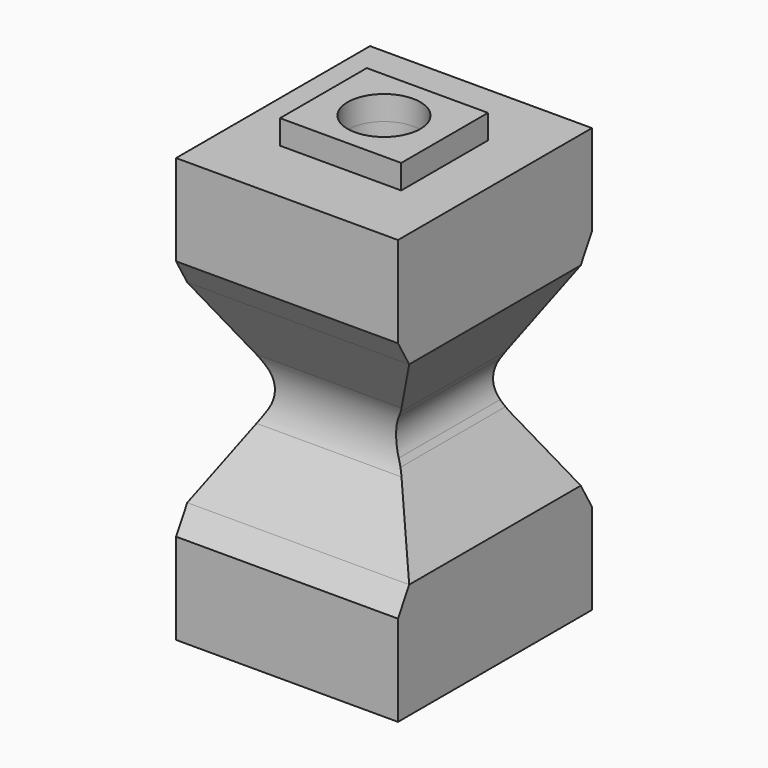
from build123d import *

# Parameters (mm, degrees)
F1_DEPTH = 10
F3_DEPTH = 18.3104010768
F5_DEPTH = 35.001
F6_W     = 10
F6_H     = 8.9491856137
F6_R     = 3
F7_DEPTH = 2


# Not quite as in the source:
# - a pattern or mirror of a feature is missing from the dataset's text; its kind, count and spacing are read off the source's solid


with BuildPart() as f1:
    # F0 (on Front) → F1 (new body, symmetric)
    with BuildSketch(Plane.XZ):
        with BuildLine():
            Line((-3.7527767497, 1.5), (-3.4641016043, 2.0000000188))
            Line((-3.4641016043, 2.0000000188), (0, 8))
            Line((0, 8), (0, 17.5))
            Line((0, 17.5), (-18.3094010768, 17.5))
            Line((-18.3094010768, 17.5), (-18.3094010768, 8))
            Line((-18.3094010768, 8), (-14.556624327, 1.5))
            ThreePointArc((-14.556624327, 1.5), (-14.1547005384, 0), (-14.556624327, -1.5))
            Line((-14.556624327, -1.5), (-18.3094010768, -8))
            Line((-18.3094010768, -8), (-18.3094010768, -17.5))
            Line((-18.3094010768, -17.5), (0, -17.5))
            Line((0, -17.5), (0, -8))
            Line((0, -8), (-3.4641016187, -1.9999999939))
            Line((-3.4641016187, -1.9999999939), (-3.7527767497, -1.5))
            ThreePointArc((-3.7527767497, -1.5), (-4.1547005384, 0), (-3.7527767497, 1.5))
        make_face()
    extrude(amount=F1_DEPTH, both=True)

    # F2 (on Right) → F3 (cut, through all)
    with BuildSketch(Plane.YZ):
        with BuildLine():
            ThreePointArc((-6.7017059222, 0), (-7.2468927023, 4.1411047244), (-8.8452994645, 8.0000000049))
            Line((-8.8452994645, 8), (-10, 8))
            Line((-10, 8), (-10, 1.5))
            Line((-10, 1.5), (-10, -8))
            Line((-10, -8), (-10, -9.7296796796))
            ThreePointArc((-10, -9.7296796796), (-9.3945168749, -8.8836208643), (-8.8452995254, -8.0000001104))
            ThreePointArc((-8.8452995254, -8.0000001104), (-7.246892718, -4.1411047832), (-6.7017059222, 0))
        make_face()
        with BuildLine():
            ThreePointArc((-8.8452994645, 8.0000000049), (-9.3945168411, 8.8836208136), (-10, 9.7296796796))
            Line((-10, 9.7296796796), (-10, 8))
            Line((-10, 8), (-8.8452994645, 8))
        make_face()
        with BuildLine():
            Line((-5.6698729811, 2.5), (-8.8452994645, 8.0000000049))
            ThreePointArc((-8.8452994645, 8.0000000049), (-7.2468927023, 4.1411047244), (-6.7017059222, 0))
            ThreePointArc((-6.7017059222, 0), (-7.246892718, -4.1411047832), (-8.8452995254, -8.0000001104))
            Line((-8.8452995254, -8.0000001104), (-5.6698729811, -2.5))
            ThreePointArc((-5.6698729811, -2.5), (-5, 0), (-5.6698729811, 2.5))
        make_face()
        with BuildLine():
            Line((-8.8452994645, 8.0000000049), (-10, 10))
            Line((-10, 10), (-10, 9.7296796796))
            ThreePointArc((-10, 9.7296796796), (-9.3945168411, 8.8836208136), (-8.8452994645, 8.0000000049))
        make_face()
        with BuildLine():
            ThreePointArc((-8.8452995254, -8.0000001104), (-9.3945168749, -8.8836208643), (-10, -9.7296796796))
            Line((-10, -9.7296796796), (-10, -10))
            Line((-10, -10), (-8.8452995254, -8.0000001104))
        make_face()
    f3 = extrude(amount=-F3_DEPTH, mode=Mode.SUBTRACT)

    # F3_copies: F3 across plane
    add(f3.mirror(Plane.ZX), mode=Mode.SUBTRACT)

    # F4 (on face) → F5 (cut, through all)
    with BuildSketch(Plane(origin=(0, 0, -17.5), x_dir=(1, 0, 0), z_dir=(0, 0, -1))):
        with BuildLine():
            Line((-11.1804351675, 2.2127808776), (-7.1289659092, -2.2127808776))
            ThreePointArc((-7.1289659092, -2.2127808776), (-6.4090490777, -1.2088829787), (-6.1547005384, 0))
            ThreePointArc((-6.1547005384, 0), (-7.9458175596, 2.7456514607), (-11.1804351675, 2.2127808776))
        make_face()
        with BuildLine():
            ThreePointArc((-11.1804351675, 2.2127808776), (-11.367481416, -2.0257346291), (-7.1289659092, -2.2127808776))
            Line((-7.1289659092, -2.2127808776), (-11.1804351675, 2.2127808776))
        make_face()
    extrude(amount=-F5_DEPTH, mode=Mode.SUBTRACT)

    # F6 (on face) → F7 (join)
    with BuildSketch(Plane.XY.offset(17.5)):
        with Locations((-9.1547005384, 0)):
            Rectangle(F6_W, F6_H)
        with Locations((-9.1547005384, 0)):
            Circle(F6_R, mode=Mode.SUBTRACT)
    extrude(amount=F7_DEPTH)


solid = f1.part
